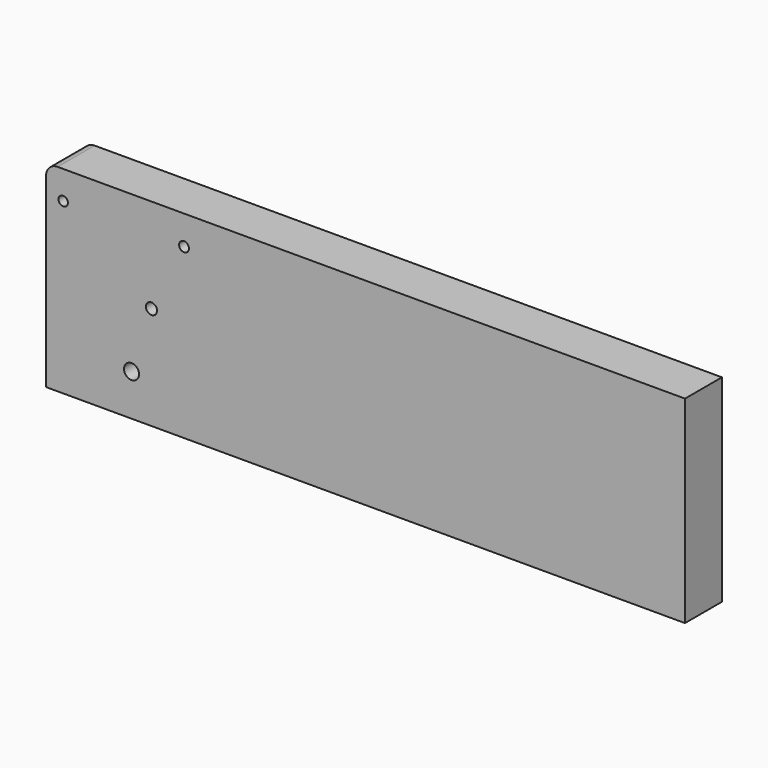
from build123d import *

# Parameters (mm, degrees)
F0_R     = 4.145299883
F0_R_2   = 2.5851912666
F0_R_3   = 3.0648919033
F0_R_4   = 2.7118286766
F1_DEPTH = 25.4
F2_DEPTH = 254


# Not quite as in the source:
# - the program builds the solid bodies; features that only make, move or delete a surface that nothing else refers to are left out


with BuildPart() as f1:
    # F0 (on Front) → F1 (new body)
    with BuildSketch(Plane.XZ):
        with BuildLine():
            Line((50.6008081138, 51.9382767379), (-40.6842338085, 51.9382767379))
            ThreePointArc((-40.6842338085, 51.9382767379), (-45.1743618691, 50.0784047985), (-47.0342338085, 45.5882767379))
            Line((-47.0342338085, 45.5882767379), (-47.0342338085, -56.842315942))
            Line((-47.0342338085, -56.842315942), (50.6008081138, -56.842315942))
            Line((50.6008081138, -56.842315942), (50.6008081138, 51.9382767379))
        make_face()
        with Locations((0, -34.0232253075)):
            Circle(F0_R, mode=Mode.SUBTRACT)
        with Locations((-37.6131273806, 36.3515801728)):
            Circle(F0_R_2, mode=Mode.SUBTRACT)
        with Locations((10.9797539189, 0)):
            Circle(F0_R_3, mode=Mode.SUBTRACT)
        with Locations((28.9033185691, 35.878714174)):
            Circle(F0_R_4, mode=Mode.SUBTRACT)
    extrude(amount=F1_DEPTH)

    # F2 (add): a face of the model
    f2_faces = [f1.faces().sort_by_distance(p)[0] for p in [
        (50.6008081138, -12.7, -2.4520196021),
    ]]
    extrude(f2_faces, amount=F2_DEPTH)


solid = f1.part
